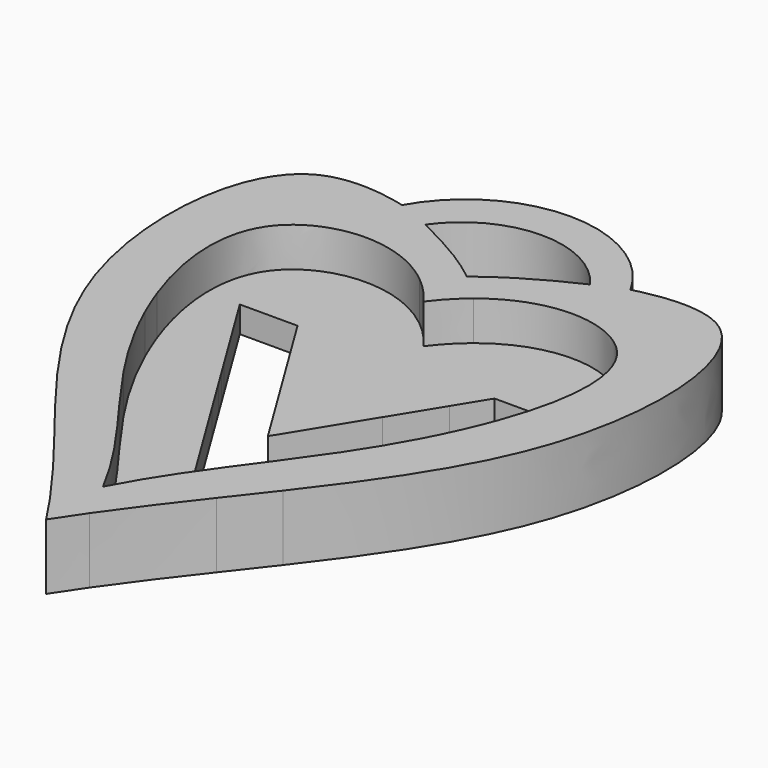
from build123d import *

# Parameters (mm, degrees)
F1_DEPTH = 3
F2_DEPTH = 1.2


with BuildPart() as f1:
    # F0 (on Top) → F1 (new body)
    with BuildSketch(Plane.XY):
        with BuildLine():
            add(Edge.make_bspline(
                [(-4.9749169396, 2.2570605233), (-5.4315886999, 2.9367985469), (-6.2390267735, 4.2240527549), (-6.9739655577, 5.6827413336), (-7.2721294197, 6.351229041)],
                knots=[0.1600128874, 0.1600128874, 0.1600128874, 0.1600128874, 0.203311187, 0.2384958301, 0.2384958301, 0.2384958301, 0.2384958301], degree=3))
            add(Edge.make_bspline(
                [(-7.2721294197, 6.351229041), (-7.4788674816, 6.8147387773), (-7.6705499156, 7.2852406632), (-7.8415947895, 7.7560973487)],
                knots=[0.2384958301, 0.2384958301, 0.2384958301, 0.2384958301, 0.262891828, 0.262891828, 0.262891828, 0.262891828], degree=3))
            add(Edge.make_bspline(
                [(-7.8415947895, 7.7560973487), (-8.7623981845, 10.290908388), (-9.4393977459, 15.6302209214), (-3.6512791674, 16.4572689664), (-1.2366444657, 14.5133787418)],
                knots=[0.262891828, 0.262891828, 0.262891828, 0.262891828, 0.3942253029, 0.5384143068, 0.5384143068, 0.5384143068, 0.5384143068], degree=3))
            add(Edge.make_bspline(
                [(0, 15.690593828), (-0.4541475038, 15.3244788933), (-0.8646901654, 14.9326448002), (-1.2366444657, 14.5133787418)],
                knots=[0.4891207725, 0.4891207725, 0.4891207725, 0.4891207725, 0.5112638272, 0.5112638272, 0.5112638272, 0.5112638272], degree=3))
            add(Edge.make_bspline(
                [(-3.6766897187, 17.8989388932), (-2.6202663938, 17.4014618162), (-1.166333928, 16.630844003), (0, 15.690593828)],
                knots=[0.4322533544, 0.4322533544, 0.4322533544, 0.4322533544, 0.4891207725, 0.4891207725, 0.4891207725, 0.4891207725], degree=3))
            add(Edge.make_bspline(
                [(-5.2704766416, 18.5644548202), (-5.2348405777, 18.5548707596), (-5.1171635403, 18.5222978976), (-5.1015113199, 18.5179293498), (-4.3735677666, 18.2271036034), (-3.6766897187, 17.8989388932)],
                knots=[0.3752902915, 0.3752902915, 0.3752902915, 0.3752902915, 0.3801303368, 0.3947403097, 0.4322533544, 0.4322533544, 0.4322533544, 0.4322533544], degree=3))
            add(Edge.make_bspline(
                [(-5.2173877822, -1.3526297811), (-7.4176426599, 1.4964237869), (-12.1799787385, 8.2048314108), (-11.3873193532, 20.0619992009), (-5.8135375277, 18.7105071022), (-5.2704766416, 18.5644548202)],
                knots=[0.0761262419, 0.0761262419, 0.0761262419, 0.0761262419, 0.171603356, 0.3015324463, 0.3752902915, 0.3752902915, 0.3752902915, 0.3752902915], degree=3))
            add(Edge.make_bspline(
                [(-4.9749169299, 2.2570605253), (-5.0764322839, 1.0820371928), (-5.1549018853, -0.1299275648), (-5.2173877716, -1.3526297784)],
                knots=[0.657103344, 0.657103344, 0.657103344, 0.657103344, 0.6891427694, 0.6891427694, 0.6891427694, 0.6891427694], degree=3))
        make_face()
        with BuildLine():
            add(Edge.make_bspline(
                [(-3.545053861, 0.2367084055), (-4.0256690115, 0.8937828722), (-4.5062005837, 1.559394591), (-4.9749169396, 2.2570605233)],
                knots=[0.1155726067, 0.1155726067, 0.1155726067, 0.1155726067, 0.1600128874, 0.1600128874, 0.1600128874, 0.1600128874], degree=3))
            add(Edge.make_bspline(
                [(-4.9749169299, 2.2570605253), (-5.0764322839, 1.0820371928), (-5.1549018853, -0.1299275648), (-5.2173877716, -1.3526297784)],
                knots=[0.657103344, 0.657103344, 0.657103344, 0.657103344, 0.6891427694, 0.6891427694, 0.6891427694, 0.6891427694], degree=3))
            add(Edge.make_bspline(
                [(-3.71718405, -3.2765240813), (-4.2206036802, -2.6317819208), (-4.7236049542, -1.9920164914), (-5.2173877822, -1.3526297811)],
                knots=[0.0546991973, 0.0546991973, 0.0546991973, 0.0546991973, 0.0761262419, 0.0761262419, 0.0761262419, 0.0761262419], degree=3))
            add(Edge.make_bspline(
                [(-3.545053871, 0.2367084032), (-3.6430205743, -0.9790737326), (-3.6986039657, -2.1657430558), (-3.7171840497, -3.2765240813)],
                knots=[0.7068125441, 0.7068125441, 0.7068125441, 0.7068125441, 0.7424399986, 0.7424399986, 0.7424399986, 0.7424399986], degree=3))
        make_face()
        with BuildLine():
            add(Edge.make_bspline(
                [(0, 15.690593828), (-0.4541475038, 15.3244788933), (-0.8646901654, 14.9326448002), (-1.2366444657, 14.5133787418)],
                knots=[0.4891207725, 0.4891207725, 0.4891207725, 0.4891207725, 0.5112638272, 0.5112638272, 0.5112638272, 0.5112638272], degree=3))
            add(Edge.make_bspline(
                [(-1.2366444657, 14.5133787418), (-0.7995835935, 14.1615249577), (-0.3826540753, 13.7318035455), (0, 13.217448597)],
                knots=[0.5384143068, 0.5384143068, 0.5384143068, 0.5384143068, 0.5645132326, 0.5645132326, 0.5645132326, 0.5645132326], degree=3))
            add(Edge.make_bspline(
                [(1.2366444657, 14.5133787418), (0.7995835935, 14.1615249577), (0.3826540753, 13.7318035455), (0, 13.217448597)],
                knots=[0.5384143068, 0.5384143068, 0.5384143068, 0.5384143068, 0.5645132326, 0.5645132326, 0.5645132326, 0.5645132326], degree=3))
            add(Edge.make_bspline(
                [(0, 15.690593828), (0.4541475038, 15.3244788933), (0.8646901654, 14.9326448002), (1.2366444657, 14.5133787418)],
                knots=[0.4891207725, 0.4891207725, 0.4891207725, 0.4891207725, 0.5112638272, 0.5112638272, 0.5112638272, 0.5112638272], degree=3))
        make_face()
        with BuildLine():
            add(Edge.make_bspline(
                [(0, -5.1301232883), (-1.0446868472, -3.1231634978), (-2.2951529848, -1.472097384), (-3.545053861, 0.2367084055)],
                knots=[0, 0, 0, 0, 0.1155726067, 0.1155726067, 0.1155726067, 0.1155726067], degree=3))
            add(Edge.make_bspline(
                [(-3.545053871, 0.2367084032), (-3.6430205743, -0.9790737326), (-3.6986039657, -2.1657430558), (-3.7171840497, -3.2765240813)],
                knots=[0.7068125441, 0.7068125441, 0.7068125441, 0.7068125441, 0.7424399986, 0.7424399986, 0.7424399986, 0.7424399986], degree=3))
            add(Edge.make_bspline(
                [(-0.909503323, -7.0283931962), (-1.8069276842, -5.738998119), (-2.762807655, -4.4988178934), (-3.71718405, -3.2765240813)],
                knots=[0.0140780844, 0.0140780844, 0.0140780844, 0.0140780844, 0.0546991973, 0.0546991973, 0.0546991973, 0.0546991973], degree=3))
            add(Edge.make_bspline(
                [(-0.909503323, -7.0283931962), (-0.6260424555, -6.4045651868), (-0.322847632, -5.7503495481), (0, -5.1301232883)],
                knots=[0.9642837062, 0.9642837062, 0.9642837062, 0.9642837062, 1, 1, 1, 1], degree=3))
        make_face()
        with BuildLine():
            add(Edge.make_bspline(
                [(3.8197797332, 17.9657974624), (2.7545346175, 17.4719466169), (1.2199446973, 16.6740627879), (0, 15.690593828)],
                knots=[0.4296394323, 0.4296394323, 0.4296394323, 0.4296394323, 0.4891207725, 0.4891207725, 0.4891207725, 0.4891207725], degree=3))
            add(Edge.make_bspline(
                [(0, 15.690593828), (0.4541475038, 15.3244788933), (0.8646901654, 14.9326448002), (1.2366444657, 14.5133787418)],
                knots=[0.4891207725, 0.4891207725, 0.4891207725, 0.4891207725, 0.5112638272, 0.5112638272, 0.5112638272, 0.5112638272], degree=3))
            add(Edge.make_bspline(
                [(7.8415947895, 7.7560973487), (8.7623981845, 10.290908388), (9.4393977459, 15.6302209214), (3.6512791674, 16.4572689664), (1.2366444657, 14.5133787418)],
                knots=[0.262891828, 0.262891828, 0.262891828, 0.262891828, 0.3942253029, 0.5384143068, 0.5384143068, 0.5384143068, 0.5384143068], degree=3))
            add(Edge.make_bspline(
                [(7.2721294197, 6.351229041), (7.4788674816, 6.8147387773), (7.6705499156, 7.2852406632), (7.8415947895, 7.7560973487)],
                knots=[0.2384958301, 0.2384958301, 0.2384958301, 0.2384958301, 0.262891828, 0.262891828, 0.262891828, 0.262891828], degree=3))
            add(Edge.make_bspline(
                [(4.9749169396, 2.2570605233), (5.4315886999, 2.9367985469), (6.2390267735, 4.2240527549), (6.9739655577, 5.6827413336), (7.2721294197, 6.351229041)],
                knots=[0.1600128874, 0.1600128874, 0.1600128874, 0.1600128874, 0.203311187, 0.2384958301, 0.2384958301, 0.2384958301, 0.2384958301], degree=3))
            add(Edge.make_bspline(
                [(4.9749169299, 2.2570605253), (5.0764322839, 1.0820371928), (5.1549018853, -0.1299275648), (5.2173877716, -1.3526297784)],
                knots=[0.657103344, 0.657103344, 0.657103344, 0.657103344, 0.6891427694, 0.6891427694, 0.6891427694, 0.6891427694], degree=3))
            add(Edge.make_bspline(
                [(5.2173877822, -1.3526297811), (7.4176426599, 1.4964237869), (12.1799787385, 8.2048314108), (11.377609767, 20.2072421577), (5.6113499273, 18.6588265968), (5.2007195954, 18.5454217718)],
                knots=[0.0761262419, 0.0761262419, 0.0761262419, 0.0761262419, 0.171603356, 0.3015324463, 0.3789548657, 0.3789548657, 0.3789548657, 0.3789548657], degree=3))
            add(Edge.make_bspline(
                [(5.2007195954, 18.5454217718), (5.1944851728, 18.5436999954), (5.1161565944, 18.5220168582), (5.1022295693, 18.5181298138), (4.4447844771, 18.2555515449), (3.8197797332, 17.9657974624)],
                knots=[0.3789548657, 0.3789548657, 0.3789548657, 0.3789548657, 0.3801303368, 0.3947403097, 0.4296394323, 0.4296394323, 0.4296394323, 0.4296394323], degree=3))
        make_face()
        with BuildLine():
            add(Edge.make_bspline(
                [(0, -5.1301232883), (1.0446868472, -3.1231634978), (2.2951529848, -1.472097384), (3.545053861, 0.2367084055)],
                knots=[0, 0, 0, 0, 0.1155726067, 0.1155726067, 0.1155726067, 0.1155726067], degree=3))
            add(Edge.make_bspline(
                [(0.909503323, -7.0283931962), (0.6260424555, -6.4045651868), (0.322847632, -5.7503495481), (0, -5.1301232883)],
                knots=[0.9642837062, 0.9642837062, 0.9642837062, 0.9642837062, 1, 1, 1, 1], degree=3))
            add(Edge.make_bspline(
                [(0.909503323, -7.0283931962), (1.8069276842, -5.738998119), (2.762807655, -4.4988178934), (3.71718405, -3.2765240813)],
                knots=[0.0140780844, 0.0140780844, 0.0140780844, 0.0140780844, 0.0546991973, 0.0546991973, 0.0546991973, 0.0546991973], degree=3))
            add(Edge.make_bspline(
                [(3.545053871, 0.2367084032), (3.6430205743, -0.9790737326), (3.6986039657, -2.1657430558), (3.7171840497, -3.2765240813)],
                knots=[0.7068125441, 0.7068125441, 0.7068125441, 0.7068125441, 0.7424399986, 0.7424399986, 0.7424399986, 0.7424399986], degree=3))
        make_face()
        with BuildLine():
            add(Edge.make_bspline(
                [(0.909503323, -7.0283931962), (0.6260424555, -6.4045651868), (0.322847632, -5.7503495481), (0, -5.1301232883)],
                knots=[0.9642837062, 0.9642837062, 0.9642837062, 0.9642837062, 1, 1, 1, 1], degree=3))
            add(Edge.make_bspline(
                [(-0.909503323, -7.0283931962), (-0.6260424555, -6.4045651868), (-0.322847632, -5.7503495481), (0, -5.1301232883)],
                knots=[0.9642837062, 0.9642837062, 0.9642837062, 0.9642837062, 1, 1, 1, 1], degree=3))
            add(Edge.make_bspline(
                [(0, -8.3880304423), (-0.2944826532, -7.928037366), (-0.5984824014, -7.4752596537), (-0.909503323, -7.0283931962)],
                knots=[0, 0, 0, 0, 0.0140780844, 0.0140780844, 0.0140780844, 0.0140780844], degree=3))
            add(Edge.make_bspline(
                [(0, -8.3880304423), (0.2944826532, -7.928037366), (0.5984824014, -7.4752596537), (0.909503323, -7.0283931962)],
                knots=[0, 0, 0, 0, 0.0140780844, 0.0140780844, 0.0140780844, 0.0140780844], degree=3))
        make_face()
        with BuildLine():
            ThreePointArc((5.2007195954, 18.5454217718), (-0.0292679208, 21.6416597117), (-5.2704766416, 18.5644548202))
            add(Edge.make_bspline(
                [(-5.2704766416, 18.5644548202), (-5.2348405777, 18.5548707596), (-5.1171635403, 18.5222978976), (-5.1015113199, 18.5179293498), (-4.3735677666, 18.2271036034), (-3.6766897187, 17.8989388932)],
                knots=[0.3752902915, 0.3752902915, 0.3752902915, 0.3752902915, 0.3801303368, 0.3947403097, 0.4322533544, 0.4322533544, 0.4322533544, 0.4322533544], degree=3))
            ThreePointArc((-3.6766897187, 17.8989388932), (0.0542828054, 19.8678802684), (3.8197797332, 17.9657974624))
            add(Edge.make_bspline(
                [(5.2007195954, 18.5454217718), (5.1944851728, 18.5436999954), (5.1161565944, 18.5220168582), (5.1022295693, 18.5181298138), (4.4447844771, 18.2555515449), (3.8197797332, 17.9657974624)],
                knots=[0.3789548657, 0.3789548657, 0.3789548657, 0.3789548657, 0.3801303368, 0.3947403097, 0.4296394323, 0.4296394323, 0.4296394323, 0.4296394323], degree=3))
        make_face()
        with BuildLine():
            add(Edge.make_bspline(
                [(3.545053861, 0.2367084055), (4.0256690115, 0.8937828722), (4.5062005837, 1.559394591), (4.9749169396, 2.2570605233)],
                knots=[0.1155726067, 0.1155726067, 0.1155726067, 0.1155726067, 0.1600128874, 0.1600128874, 0.1600128874, 0.1600128874], degree=3))
            add(Edge.make_bspline(
                [(3.545053871, 0.2367084032), (3.6430205743, -0.9790737326), (3.6986039657, -2.1657430558), (3.7171840497, -3.2765240813)],
                knots=[0.7068125441, 0.7068125441, 0.7068125441, 0.7068125441, 0.7424399986, 0.7424399986, 0.7424399986, 0.7424399986], degree=3))
            add(Edge.make_bspline(
                [(3.71718405, -3.2765240813), (4.2206036802, -2.6317819208), (4.7236049542, -1.9920164914), (5.2173877822, -1.3526297811)],
                knots=[0.0546991973, 0.0546991973, 0.0546991973, 0.0546991973, 0.0761262419, 0.0761262419, 0.0761262419, 0.0761262419], degree=3))
            add(Edge.make_bspline(
                [(4.9749169299, 2.2570605253), (5.0764322839, 1.0820371928), (5.1549018853, -0.1299275648), (5.2173877716, -1.3526297784)],
                knots=[0.657103344, 0.657103344, 0.657103344, 0.657103344, 0.6891427694, 0.6891427694, 0.6891427694, 0.6891427694], degree=3))
        make_face()
    extrude(amount=F1_DEPTH)

    # F0 (on Top) → F2 (join)
    with BuildSketch(Plane.XY):
        with BuildLine():
            add(Edge.make_bspline(
                [(-4.9749169396, 2.2570605233), (-5.4315886999, 2.9367985469), (-6.2390267735, 4.2240527549), (-6.9739655577, 5.6827413336), (-7.2721294197, 6.351229041)],
                knots=[0.1600128874, 0.1600128874, 0.1600128874, 0.1600128874, 0.203311187, 0.2384958301, 0.2384958301, 0.2384958301, 0.2384958301], degree=3))
            add(Edge.make_bspline(
                [(-7.2721294197, 6.351229041), (-7.4788674816, 6.8147387773), (-7.6705499156, 7.2852406632), (-7.8415947895, 7.7560973487)],
                knots=[0.2384958301, 0.2384958301, 0.2384958301, 0.2384958301, 0.262891828, 0.262891828, 0.262891828, 0.262891828], degree=3))
            add(Edge.make_bspline(
                [(-7.8415947895, 7.7560973487), (-8.7623981845, 10.290908388), (-9.4393977459, 15.6302209214), (-3.6512791674, 16.4572689664), (-1.2366444657, 14.5133787418)],
                knots=[0.262891828, 0.262891828, 0.262891828, 0.262891828, 0.3942253029, 0.5384143068, 0.5384143068, 0.5384143068, 0.5384143068], degree=3))
            add(Edge.make_bspline(
                [(0, 15.690593828), (-0.4541475038, 15.3244788933), (-0.8646901654, 14.9326448002), (-1.2366444657, 14.5133787418)],
                knots=[0.4891207725, 0.4891207725, 0.4891207725, 0.4891207725, 0.5112638272, 0.5112638272, 0.5112638272, 0.5112638272], degree=3))
            add(Edge.make_bspline(
                [(-3.6766897187, 17.8989388932), (-2.6202663938, 17.4014618162), (-1.166333928, 16.630844003), (0, 15.690593828)],
                knots=[0.4322533544, 0.4322533544, 0.4322533544, 0.4322533544, 0.4891207725, 0.4891207725, 0.4891207725, 0.4891207725], degree=3))
            add(Edge.make_bspline(
                [(-5.2704766416, 18.5644548202), (-5.2348405777, 18.5548707596), (-5.1171635403, 18.5222978976), (-5.1015113199, 18.5179293498), (-4.3735677666, 18.2271036034), (-3.6766897187, 17.8989388932)],
                knots=[0.3752902915, 0.3752902915, 0.3752902915, 0.3752902915, 0.3801303368, 0.3947403097, 0.4322533544, 0.4322533544, 0.4322533544, 0.4322533544], degree=3))
            add(Edge.make_bspline(
                [(-5.2173877822, -1.3526297811), (-7.4176426599, 1.4964237869), (-12.1799787385, 8.2048314108), (-11.3873193532, 20.0619992009), (-5.8135375277, 18.7105071022), (-5.2704766416, 18.5644548202)],
                knots=[0.0761262419, 0.0761262419, 0.0761262419, 0.0761262419, 0.171603356, 0.3015324463, 0.3752902915, 0.3752902915, 0.3752902915, 0.3752902915], degree=3))
            add(Edge.make_bspline(
                [(-4.9749169299, 2.2570605253), (-5.0764322839, 1.0820371928), (-5.1549018853, -0.1299275648), (-5.2173877716, -1.3526297784)],
                knots=[0.657103344, 0.657103344, 0.657103344, 0.657103344, 0.6891427694, 0.6891427694, 0.6891427694, 0.6891427694], degree=3))
        make_face()
        with BuildLine():
            Line((-4.4866587821, 6.351229041), (-7.2721294197, 6.351229041))
            add(Edge.make_bspline(
                [(-4.9749169396, 2.2570605233), (-5.4315886999, 2.9367985469), (-6.2390267735, 4.2240527549), (-6.9739655577, 5.6827413336), (-7.2721294197, 6.351229041)],
                knots=[0.1600128874, 0.1600128874, 0.1600128874, 0.1600128874, 0.203311187, 0.2384958301, 0.2384958301, 0.2384958301, 0.2384958301], degree=3))
            add(Edge.make_bspline(
                [(-4.4866587821, 6.351229041), (-4.6924126216, 5.0735396285), (-4.8508702833, 3.6928798215), (-4.9749169299, 2.2570605253)],
                knots=[0.617952781, 0.617952781, 0.617952781, 0.617952781, 0.657103344, 0.657103344, 0.657103344, 0.657103344], degree=3))
        make_face()
        with BuildLine():
            add(Edge.make_bspline(
                [(-7.2721294197, 6.351229041), (-7.4788674816, 6.8147387773), (-7.6705499156, 7.2852406632), (-7.8415947895, 7.7560973487)],
                knots=[0.2384958301, 0.2384958301, 0.2384958301, 0.2384958301, 0.262891828, 0.262891828, 0.262891828, 0.262891828], degree=3))
            Line((-7.2721294197, 6.351229041), (-4.4866587821, 6.351229041))
            add(Edge.make_bspline(
                [(-4.3596876264, 7.0926991318), (-4.3702142327, 7.0348686428), (-4.4139730933, 6.7909039185), (-4.4558282844, 6.5426801493), (-4.4866587821, 6.351229041)],
                knots=[0.6102538131, 0.6102538131, 0.6102538131, 0.6102538131, 0.6120863954, 0.617952781, 0.617952781, 0.617952781, 0.617952781], degree=3))
            Line((-4.3596876264, 7.0926991318), (-4.7674603154, 7.7560973487))
            Line((-4.7674603154, 7.7560973487), (-7.8415947895, 7.7560973487))
        make_face()
        with BuildLine():
            add(Edge.make_bspline(
                [(-7.8415947895, 7.7560973487), (-8.7623981845, 10.290908388), (-9.4393977459, 15.6302209214), (-3.6512791674, 16.4572689664), (-1.2366444657, 14.5133787418)],
                knots=[0.262891828, 0.262891828, 0.262891828, 0.262891828, 0.3942253029, 0.5384143068, 0.5384143068, 0.5384143068, 0.5384143068], degree=3))
            Line((-7.8415947895, 7.7560973487), (-4.7674603154, 7.7560973487))
            Line((-4.7674603154, 7.7560973487), (-7.1526595965, 11.6365361141))
            Line((-7.1526595965, 11.6365361141), (-4.5090120843, 11.6365361141))
            Line((-4.5090120843, 11.6365361141), (-3.6085880649, 10.1716521113))
            add(Edge.make_bspline(
                [(-1.2366444657, 14.5133787418), (-2.3069834299, 13.3068950462), (-3.0577863597, 11.8732573307), (-3.6085880649, 10.1716521113)],
                knots=[0.5112638272, 0.5112638272, 0.5112638272, 0.5112638272, 0.5749828761, 0.5749828761, 0.5749828761, 0.5749828761], degree=3))
        make_face()
        with BuildLine():
            add(Edge.make_bspline(
                [(-4.4866587821, 6.351229041), (-4.6924126216, 5.0735396285), (-4.8508702833, 3.6928798215), (-4.9749169299, 2.2570605253)],
                knots=[0.617952781, 0.617952781, 0.617952781, 0.617952781, 0.657103344, 0.657103344, 0.657103344, 0.657103344], degree=3))
            add(Edge.make_bspline(
                [(-3.545053861, 0.2367084055), (-4.0256690115, 0.8937828722), (-4.5062005837, 1.559394591), (-4.9749169396, 2.2570605233)],
                knots=[0.1155726067, 0.1155726067, 0.1155726067, 0.1155726067, 0.1600128874, 0.1600128874, 0.1600128874, 0.1600128874], degree=3))
            add(Edge.make_bspline(
                [(-2.9700763494, 4.8319649824), (-3.2346608472, 3.3154483148), (-3.4228381988, 1.7534240415), (-3.545053871, 0.2367084032)],
                knots=[0.6623664909, 0.6623664909, 0.6623664909, 0.6623664909, 0.7068125441, 0.7068125441, 0.7068125441, 0.7068125441], degree=3))
            Line((-2.9700763494, 4.8319649824), (-3.9039262977, 6.351229041))
            Line((-3.9039262977, 6.351229041), (-4.4866587821, 6.351229041))
        make_face()
        with BuildLine():
            add(Edge.make_bspline(
                [(-3.545053861, 0.2367084055), (-4.0256690115, 0.8937828722), (-4.5062005837, 1.559394591), (-4.9749169396, 2.2570605233)],
                knots=[0.1155726067, 0.1155726067, 0.1155726067, 0.1155726067, 0.1600128874, 0.1600128874, 0.1600128874, 0.1600128874], degree=3))
            add(Edge.make_bspline(
                [(-4.9749169299, 2.2570605253), (-5.0764322839, 1.0820371928), (-5.1549018853, -0.1299275648), (-5.2173877716, -1.3526297784)],
                knots=[0.657103344, 0.657103344, 0.657103344, 0.657103344, 0.6891427694, 0.6891427694, 0.6891427694, 0.6891427694], degree=3))
            add(Edge.make_bspline(
                [(-3.71718405, -3.2765240813), (-4.2206036802, -2.6317819208), (-4.7236049542, -1.9920164914), (-5.2173877822, -1.3526297811)],
                knots=[0.0546991973, 0.0546991973, 0.0546991973, 0.0546991973, 0.0761262419, 0.0761262419, 0.0761262419, 0.0761262419], degree=3))
            add(Edge.make_bspline(
                [(-3.545053871, 0.2367084032), (-3.6430205743, -0.9790737326), (-3.6986039657, -2.1657430558), (-3.7171840497, -3.2765240813)],
                knots=[0.7068125441, 0.7068125441, 0.7068125441, 0.7068125441, 0.7424399986, 0.7424399986, 0.7424399986, 0.7424399986], degree=3))
        make_face()
        with BuildLine():
            add(Edge.make_bspline(
                [(-4.3596876264, 7.0926991318), (-4.3702142327, 7.0348686428), (-4.4139730933, 6.7909039185), (-4.4558282844, 6.5426801493), (-4.4866587821, 6.351229041)],
                knots=[0.6102538131, 0.6102538131, 0.6102538131, 0.6102538131, 0.6120863954, 0.617952781, 0.617952781, 0.617952781, 0.617952781], degree=3))
            Line((-4.4866587821, 6.351229041), (-3.9039262977, 6.351229041))
            Line((-3.9039262977, 6.351229041), (-4.3596876264, 7.0926991318))
        make_face()
        with BuildLine():
            add(Edge.make_bspline(
                [(0, 15.690593828), (-0.4541475038, 15.3244788933), (-0.8646901654, 14.9326448002), (-1.2366444657, 14.5133787418)],
                knots=[0.4891207725, 0.4891207725, 0.4891207725, 0.4891207725, 0.5112638272, 0.5112638272, 0.5112638272, 0.5112638272], degree=3))
            add(Edge.make_bspline(
                [(-1.2366444657, 14.5133787418), (-0.7995835935, 14.1615249577), (-0.3826540753, 13.7318035455), (0, 13.217448597)],
                knots=[0.5384143068, 0.5384143068, 0.5384143068, 0.5384143068, 0.5645132326, 0.5645132326, 0.5645132326, 0.5645132326], degree=3))
            add(Edge.make_bspline(
                [(1.2366444657, 14.5133787418), (0.7995835935, 14.1615249577), (0.3826540753, 13.7318035455), (0, 13.217448597)],
                knots=[0.5384143068, 0.5384143068, 0.5384143068, 0.5384143068, 0.5645132326, 0.5645132326, 0.5645132326, 0.5645132326], degree=3))
            add(Edge.make_bspline(
                [(0, 15.690593828), (0.4541475038, 15.3244788933), (0.8646901654, 14.9326448002), (1.2366444657, 14.5133787418)],
                knots=[0.4891207725, 0.4891207725, 0.4891207725, 0.4891207725, 0.5112638272, 0.5112638272, 0.5112638272, 0.5112638272], degree=3))
        make_face()
        with BuildLine():
            add(Edge.make_bspline(
                [(-1.2366444657, 14.5133787418), (-0.7995835935, 14.1615249577), (-0.3826540753, 13.7318035455), (0, 13.217448597)],
                knots=[0.5384143068, 0.5384143068, 0.5384143068, 0.5384143068, 0.5645132326, 0.5645132326, 0.5645132326, 0.5645132326], degree=3))
            add(Edge.make_bspline(
                [(-1.2366444657, 14.5133787418), (-2.3069834299, 13.3068950462), (-3.0577863597, 11.8732573307), (-3.6085880649, 10.1716521113)],
                knots=[0.5112638272, 0.5112638272, 0.5112638272, 0.5112638272, 0.5749828761, 0.5749828761, 0.5749828761, 0.5749828761], degree=3))
            Line((-3.6085880649, 10.1716521113), (-2.2757587321, 8.0032955083))
            add(Edge.make_bspline(
                [(0, 13.217448597), (-0.9654520873, 11.9197097494), (-1.7127156823, 10.0832159765), (-2.2757587321, 8.0032955083)],
                knots=[0.5645132326, 0.5645132326, 0.5645132326, 0.5645132326, 0.6303619037, 0.6303619037, 0.6303619037, 0.6303619037], degree=3))
        make_face()
        with BuildLine():
            add(Edge.make_bspline(
                [(-2.9700763494, 4.8319649824), (-3.2346608472, 3.3154483148), (-3.4228381988, 1.7534240415), (-3.545053871, 0.2367084032)],
                knots=[0.6623664909, 0.6623664909, 0.6623664909, 0.6623664909, 0.7068125441, 0.7068125441, 0.7068125441, 0.7068125441], degree=3))
            add(Edge.make_bspline(
                [(0, -5.1301232883), (-1.0446868472, -3.1231634978), (-2.2951529848, -1.472097384), (-3.545053861, 0.2367084055)],
                knots=[0, 0, 0, 0, 0.1155726067, 0.1155726067, 0.1155726067, 0.1155726067], degree=3))
            add(Edge.make_bspline(
                [(0, -5.1301232883), (1.0446868472, -3.1231634978), (2.2951529848, -1.472097384), (3.545053861, 0.2367084055)],
                knots=[0, 0, 0, 0, 0.1155726067, 0.1155726067, 0.1155726067, 0.1155726067], degree=3))
            add(Edge.make_bspline(
                [(2.9700763494, 4.8319649824), (3.2346608472, 3.3154483148), (3.4228381988, 1.7534240415), (3.545053871, 0.2367084032)],
                knots=[0.6623664909, 0.6623664909, 0.6623664909, 0.6623664909, 0.7068125441, 0.7068125441, 0.7068125441, 0.7068125441], degree=3))
            Line((2.9700763494, 4.8319649824), (0, 0))
            Line((0, 0), (-2.9700763494, 4.8319649824))
        make_face()
        with BuildLine():
            add(Edge.make_bspline(
                [(1.2366444657, 14.5133787418), (0.7995835935, 14.1615249577), (0.3826540753, 13.7318035455), (0, 13.217448597)],
                knots=[0.5384143068, 0.5384143068, 0.5384143068, 0.5384143068, 0.5645132326, 0.5645132326, 0.5645132326, 0.5645132326], degree=3))
            add(Edge.make_bspline(
                [(0, 13.217448597), (0.9654520873, 11.9197097494), (1.7127156823, 10.0832159765), (2.2757587321, 8.0032955083)],
                knots=[0.5645132326, 0.5645132326, 0.5645132326, 0.5645132326, 0.6303619037, 0.6303619037, 0.6303619037, 0.6303619037], degree=3))
            Line((2.2757587321, 8.0032955083), (3.6085880649, 10.1716521113))
            add(Edge.make_bspline(
                [(1.2366444657, 14.5133787418), (2.3069834299, 13.3068950462), (3.0577863597, 11.8732573307), (3.6085880649, 10.1716521113)],
                knots=[0.5112638272, 0.5112638272, 0.5112638272, 0.5112638272, 0.5749828761, 0.5749828761, 0.5749828761, 0.5749828761], degree=3))
        make_face()
        with BuildLine():
            add(Edge.make_bspline(
                [(0, 13.217448597), (0.9654520873, 11.9197097494), (1.7127156823, 10.0832159765), (2.2757587321, 8.0032955083)],
                knots=[0.5645132326, 0.5645132326, 0.5645132326, 0.5645132326, 0.6303619037, 0.6303619037, 0.6303619037, 0.6303619037], degree=3))
            add(Edge.make_bspline(
                [(0, 13.217448597), (-0.9654520873, 11.9197097494), (-1.7127156823, 10.0832159765), (-2.2757587321, 8.0032955083)],
                knots=[0.5645132326, 0.5645132326, 0.5645132326, 0.5645132326, 0.6303619037, 0.6303619037, 0.6303619037, 0.6303619037], degree=3))
            Line((-2.2757587321, 8.0032955083), (0, 4.3009036476))
            Line((0, 4.3009036476), (2.2757587321, 8.0032955083))
        make_face()
        with BuildLine():
            add(Edge.make_bspline(
                [(3.8197797332, 17.9657974624), (2.7545346175, 17.4719466169), (1.2199446973, 16.6740627879), (0, 15.690593828)],
                knots=[0.4296394323, 0.4296394323, 0.4296394323, 0.4296394323, 0.4891207725, 0.4891207725, 0.4891207725, 0.4891207725], degree=3))
            add(Edge.make_bspline(
                [(0, 15.690593828), (0.4541475038, 15.3244788933), (0.8646901654, 14.9326448002), (1.2366444657, 14.5133787418)],
                knots=[0.4891207725, 0.4891207725, 0.4891207725, 0.4891207725, 0.5112638272, 0.5112638272, 0.5112638272, 0.5112638272], degree=3))
            add(Edge.make_bspline(
                [(7.8415947895, 7.7560973487), (8.7623981845, 10.290908388), (9.4393977459, 15.6302209214), (3.6512791674, 16.4572689664), (1.2366444657, 14.5133787418)],
                knots=[0.262891828, 0.262891828, 0.262891828, 0.262891828, 0.3942253029, 0.5384143068, 0.5384143068, 0.5384143068, 0.5384143068], degree=3))
            add(Edge.make_bspline(
                [(7.2721294197, 6.351229041), (7.4788674816, 6.8147387773), (7.6705499156, 7.2852406632), (7.8415947895, 7.7560973487)],
                knots=[0.2384958301, 0.2384958301, 0.2384958301, 0.2384958301, 0.262891828, 0.262891828, 0.262891828, 0.262891828], degree=3))
            add(Edge.make_bspline(
                [(4.9749169396, 2.2570605233), (5.4315886999, 2.9367985469), (6.2390267735, 4.2240527549), (6.9739655577, 5.6827413336), (7.2721294197, 6.351229041)],
                knots=[0.1600128874, 0.1600128874, 0.1600128874, 0.1600128874, 0.203311187, 0.2384958301, 0.2384958301, 0.2384958301, 0.2384958301], degree=3))
            add(Edge.make_bspline(
                [(4.9749169299, 2.2570605253), (5.0764322839, 1.0820371928), (5.1549018853, -0.1299275648), (5.2173877716, -1.3526297784)],
                knots=[0.657103344, 0.657103344, 0.657103344, 0.657103344, 0.6891427694, 0.6891427694, 0.6891427694, 0.6891427694], degree=3))
            add(Edge.make_bspline(
                [(5.2173877822, -1.3526297811), (7.4176426599, 1.4964237869), (12.1799787385, 8.2048314108), (11.377609767, 20.2072421577), (5.6113499273, 18.6588265968), (5.2007195954, 18.5454217718)],
                knots=[0.0761262419, 0.0761262419, 0.0761262419, 0.0761262419, 0.171603356, 0.3015324463, 0.3789548657, 0.3789548657, 0.3789548657, 0.3789548657], degree=3))
            add(Edge.make_bspline(
                [(5.2007195954, 18.5454217718), (5.1944851728, 18.5436999954), (5.1161565944, 18.5220168582), (5.1022295693, 18.5181298138), (4.4447844771, 18.2555515449), (3.8197797332, 17.9657974624)],
                knots=[0.3789548657, 0.3789548657, 0.3789548657, 0.3789548657, 0.3801303368, 0.3947403097, 0.4296394323, 0.4296394323, 0.4296394323, 0.4296394323], degree=3))
        make_face()
        with BuildLine():
            add(Edge.make_bspline(
                [(0, -5.1301232883), (1.0446868472, -3.1231634978), (2.2951529848, -1.472097384), (3.545053861, 0.2367084055)],
                knots=[0, 0, 0, 0, 0.1155726067, 0.1155726067, 0.1155726067, 0.1155726067], degree=3))
            add(Edge.make_bspline(
                [(0.909503323, -7.0283931962), (0.6260424555, -6.4045651868), (0.322847632, -5.7503495481), (0, -5.1301232883)],
                knots=[0.9642837062, 0.9642837062, 0.9642837062, 0.9642837062, 1, 1, 1, 1], degree=3))
            add(Edge.make_bspline(
                [(0.909503323, -7.0283931962), (1.8069276842, -5.738998119), (2.762807655, -4.4988178934), (3.71718405, -3.2765240813)],
                knots=[0.0140780844, 0.0140780844, 0.0140780844, 0.0140780844, 0.0546991973, 0.0546991973, 0.0546991973, 0.0546991973], degree=3))
            add(Edge.make_bspline(
                [(3.545053871, 0.2367084032), (3.6430205743, -0.9790737326), (3.6986039657, -2.1657430558), (3.7171840497, -3.2765240813)],
                knots=[0.7068125441, 0.7068125441, 0.7068125441, 0.7068125441, 0.7424399986, 0.7424399986, 0.7424399986, 0.7424399986], degree=3))
        make_face()
        with BuildLine():
            add(Edge.make_bspline(
                [(0.909503323, -7.0283931962), (0.6260424555, -6.4045651868), (0.322847632, -5.7503495481), (0, -5.1301232883)],
                knots=[0.9642837062, 0.9642837062, 0.9642837062, 0.9642837062, 1, 1, 1, 1], degree=3))
            add(Edge.make_bspline(
                [(-0.909503323, -7.0283931962), (-0.6260424555, -6.4045651868), (-0.322847632, -5.7503495481), (0, -5.1301232883)],
                knots=[0.9642837062, 0.9642837062, 0.9642837062, 0.9642837062, 1, 1, 1, 1], degree=3))
            add(Edge.make_bspline(
                [(0, -8.3880304423), (-0.2944826532, -7.928037366), (-0.5984824014, -7.4752596537), (-0.909503323, -7.0283931962)],
                knots=[0, 0, 0, 0, 0.0140780844, 0.0140780844, 0.0140780844, 0.0140780844], degree=3))
            add(Edge.make_bspline(
                [(0, -8.3880304423), (0.2944826532, -7.928037366), (0.5984824014, -7.4752596537), (0.909503323, -7.0283931962)],
                knots=[0, 0, 0, 0, 0.0140780844, 0.0140780844, 0.0140780844, 0.0140780844], degree=3))
        make_face()
        with BuildLine():
            add(Edge.make_bspline(
                [(7.8415947895, 7.7560973487), (8.7623981845, 10.290908388), (9.4393977459, 15.6302209214), (3.6512791674, 16.4572689664), (1.2366444657, 14.5133787418)],
                knots=[0.262891828, 0.262891828, 0.262891828, 0.262891828, 0.3942253029, 0.5384143068, 0.5384143068, 0.5384143068, 0.5384143068], degree=3))
            add(Edge.make_bspline(
                [(1.2366444657, 14.5133787418), (2.3069834299, 13.3068950462), (3.0577863597, 11.8732573307), (3.6085880649, 10.1716521113)],
                knots=[0.5112638272, 0.5112638272, 0.5112638272, 0.5112638272, 0.5749828761, 0.5749828761, 0.5749828761, 0.5749828761], degree=3))
            Line((3.6085880649, 10.1716521113), (4.5090120843, 11.6365361141))
            Line((4.5090120843, 11.6365361141), (7.1526595965, 11.6365361141))
            Line((7.1526595965, 11.6365361141), (4.7674603154, 7.7560973487))
            Line((4.7674603154, 7.7560973487), (7.8415947895, 7.7560973487))
        make_face()
        with BuildLine():
            add(Edge.make_bspline(
                [(3.545053861, 0.2367084055), (4.0256690115, 0.8937828722), (4.5062005837, 1.559394591), (4.9749169396, 2.2570605233)],
                knots=[0.1155726067, 0.1155726067, 0.1155726067, 0.1155726067, 0.1600128874, 0.1600128874, 0.1600128874, 0.1600128874], degree=3))
            add(Edge.make_bspline(
                [(3.545053871, 0.2367084032), (3.6430205743, -0.9790737326), (3.6986039657, -2.1657430558), (3.7171840497, -3.2765240813)],
                knots=[0.7068125441, 0.7068125441, 0.7068125441, 0.7068125441, 0.7424399986, 0.7424399986, 0.7424399986, 0.7424399986], degree=3))
            add(Edge.make_bspline(
                [(3.71718405, -3.2765240813), (4.2206036802, -2.6317819208), (4.7236049542, -1.9920164914), (5.2173877822, -1.3526297811)],
                knots=[0.0546991973, 0.0546991973, 0.0546991973, 0.0546991973, 0.0761262419, 0.0761262419, 0.0761262419, 0.0761262419], degree=3))
            add(Edge.make_bspline(
                [(4.9749169299, 2.2570605253), (5.0764322839, 1.0820371928), (5.1549018853, -0.1299275648), (5.2173877716, -1.3526297784)],
                knots=[0.657103344, 0.657103344, 0.657103344, 0.657103344, 0.6891427694, 0.6891427694, 0.6891427694, 0.6891427694], degree=3))
        make_face()
        with BuildLine():
            add(Edge.make_bspline(
                [(2.9700763494, 4.8319649824), (3.2346608472, 3.3154483148), (3.4228381988, 1.7534240415), (3.545053871, 0.2367084032)],
                knots=[0.6623664909, 0.6623664909, 0.6623664909, 0.6623664909, 0.7068125441, 0.7068125441, 0.7068125441, 0.7068125441], degree=3))
            add(Edge.make_bspline(
                [(3.545053861, 0.2367084055), (4.0256690115, 0.8937828722), (4.5062005837, 1.559394591), (4.9749169396, 2.2570605233)],
                knots=[0.1155726067, 0.1155726067, 0.1155726067, 0.1155726067, 0.1600128874, 0.1600128874, 0.1600128874, 0.1600128874], degree=3))
            add(Edge.make_bspline(
                [(4.4866587821, 6.351229041), (4.6924126216, 5.0735396285), (4.8508702833, 3.6928798215), (4.9749169299, 2.2570605253)],
                knots=[0.617952781, 0.617952781, 0.617952781, 0.617952781, 0.657103344, 0.657103344, 0.657103344, 0.657103344], degree=3))
            Line((4.4866587821, 6.351229041), (3.9039262977, 6.351229041))
            Line((3.9039262977, 6.351229041), (2.9700763494, 4.8319649824))
        make_face()
        with BuildLine():
            add(Edge.make_bspline(
                [(7.2721294197, 6.351229041), (7.4788674816, 6.8147387773), (7.6705499156, 7.2852406632), (7.8415947895, 7.7560973487)],
                knots=[0.2384958301, 0.2384958301, 0.2384958301, 0.2384958301, 0.262891828, 0.262891828, 0.262891828, 0.262891828], degree=3))
            Line((7.8415947895, 7.7560973487), (4.7674603154, 7.7560973487))
            Line((4.7674603154, 7.7560973487), (4.3596876264, 7.0926991318))
            add(Edge.make_bspline(
                [(4.3596876264, 7.0926991318), (4.3702142327, 7.0348686428), (4.4139730933, 6.7909039185), (4.4558282844, 6.5426801493), (4.4866587821, 6.351229041)],
                knots=[0.6102538131, 0.6102538131, 0.6102538131, 0.6102538131, 0.6120863954, 0.617952781, 0.617952781, 0.617952781, 0.617952781], degree=3))
            Line((4.4866587821, 6.351229041), (7.2721294197, 6.351229041))
        make_face()
        with BuildLine():
            add(Edge.make_bspline(
                [(4.4866587821, 6.351229041), (4.6924126216, 5.0735396285), (4.8508702833, 3.6928798215), (4.9749169299, 2.2570605253)],
                knots=[0.617952781, 0.617952781, 0.617952781, 0.617952781, 0.657103344, 0.657103344, 0.657103344, 0.657103344], degree=3))
            add(Edge.make_bspline(
                [(4.9749169396, 2.2570605233), (5.4315886999, 2.9367985469), (6.2390267735, 4.2240527549), (6.9739655577, 5.6827413336), (7.2721294197, 6.351229041)],
                knots=[0.1600128874, 0.1600128874, 0.1600128874, 0.1600128874, 0.203311187, 0.2384958301, 0.2384958301, 0.2384958301, 0.2384958301], degree=3))
            Line((7.2721294197, 6.351229041), (4.4866587821, 6.351229041))
        make_face()
        with BuildLine():
            Line((4.3596876264, 7.0926991318), (3.9039262977, 6.351229041))
            Line((3.9039262977, 6.351229041), (4.4866587821, 6.351229041))
            add(Edge.make_bspline(
                [(4.3596876264, 7.0926991318), (4.3702142327, 7.0348686428), (4.4139730933, 6.7909039185), (4.4558282844, 6.5426801493), (4.4866587821, 6.351229041)],
                knots=[0.6102538131, 0.6102538131, 0.6102538131, 0.6102538131, 0.6120863954, 0.617952781, 0.617952781, 0.617952781, 0.617952781], degree=3))
        make_face()
    extrude(amount=F2_DEPTH)


solid = f1.part
